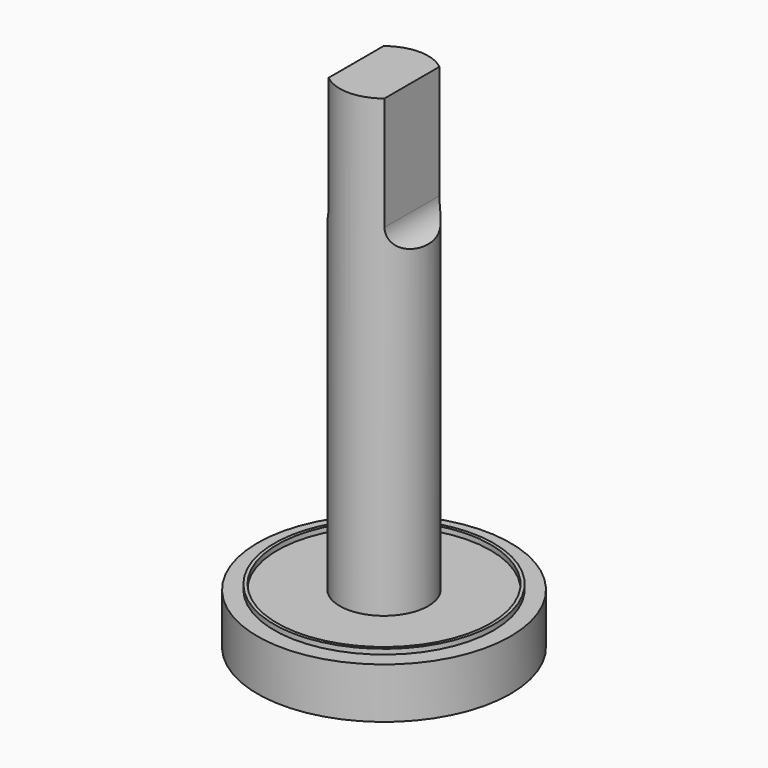
from build123d import *

# Parameters (mm, degrees)
F0_R     = 10
F0_R_2   = 3.5
F1_DEPTH = 4
F2_DEPTH = 40
F3_R     = 8.6820439201
F3_R_2   = 8.4287358905
F4_DEPTH = 0.4
F5_W     = 3.9470982738
F5_H     = 10.0623220205
F6_DEPTH = 12.5


# Not quite as in the source:
# - a feature names something its author has since deleted; it is built from what else it names


with BuildPart() as f1:
    # F0 (on Top) → F1 (new body)
    with BuildSketch(Plane.XY):
        Circle(F0_R)
        Circle(F0_R_2, mode=Mode.SUBTRACT)
        Circle(F0_R_2)
    extrude(amount=F1_DEPTH)


with BuildPart() as f2:
    # F0 (on Top) → F2 (new body)
    with BuildSketch(Plane.XY):
        Circle(F0_R_2)
    extrude(amount=F2_DEPTH)

    # F5 (on Front) → F6 (cut, symmetric)
    with BuildSketch(Plane.XZ):
        with Locations((4.183649784, 36.0617563128)):
            Rectangle(F5_W, F5_H)
        with BuildLine():
            Line((6.1571989208, 31.0305953026), (2.2101006471, 31.0305953026))
            ThreePointArc((2.2101006471, 31.0305953026), (4.183649784, 29.0570461657), (6.1571989208, 31.0305953026))
        make_face()
        with Locations((-4.183649784, 36.0617563128)):
            Rectangle(F5_W, F5_H)
        with BuildLine():
            ThreePointArc((-6.1571989208, 31.0305953026), (-4.183649784, 29.0570461657), (-2.2101006471, 31.0305953026))
            Line((-2.2101006471, 31.0305953026), (-6.1571989208, 31.0305953026))
        make_face()
    extrude(amount=F6_DEPTH, both=True, mode=Mode.SUBTRACT)


with BuildPart() as f4:
    # F3 (on face) → F4 (new body)
    with BuildSketch(Plane.XY.offset(4)):
        Circle(F3_R)
        Circle(F3_R_2, mode=Mode.SUBTRACT)
    extrude(amount=F4_DEPTH)


solid = Compound([f1.part, f2.part, f4.part])
